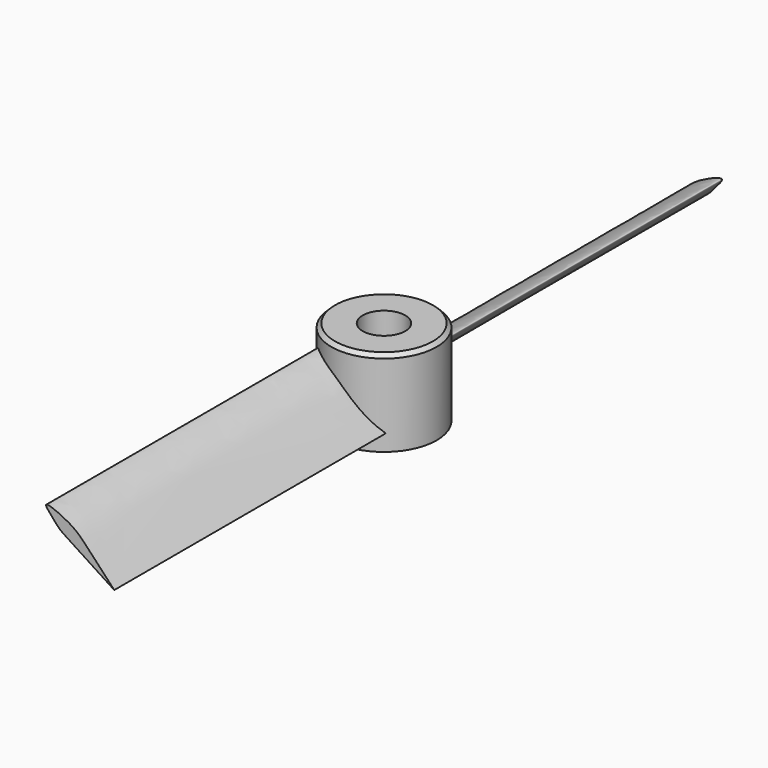
from build123d import *

# Parameters (mm, degrees)
F0_R     = 7.05
F0_R_2   = 2.85
F1_DEPTH = 11.5
F3_DEPTH = 50.8
F4_R     = 5
F6_DEPTH = 50.8
F7_R     = 5
F8_DEPTH = 25
F9_SIZE  = 0.5


# Not quite as in the source:
# - a feature names something its author has since deleted; it is built from what else it names


with BuildPart() as f1:
    # F0 (on Top) → F1 (new body)
    with BuildSketch(Plane.XY):
        Circle(F0_R)
        Circle(F0_R_2, mode=Mode.SUBTRACT)
        Circle(F0_R_2)
    extrude(amount=F1_DEPTH)

    # F2 (on Front) → F3 (join)
    with BuildSketch(Plane.XZ):
        with BuildLine():
            add(Edge.make_bspline(
                [(-2.8507792313, 7.0072189362), (-3.7405771521, 8.1520514624), (-5.7662751539, 10.0693319158), (-1.5520604506, 8.3439902136), (0.1962566258, 6.9176895133), (2.3983110105, 4.4577370851), (3.828236793, 2.9490531221), (4.5479491008, 2.1968713324)],
                knots=[0, 0, 0, 0, 0.1977876363, 0.3919769243, 0.5835513721, 0.7917756861, 1, 1, 1, 1], degree=3))
            Line((-2.8507792313, 7.0072189362), (4.5479491008, 2.1968713324))
        make_face()
    extrude(amount=F3_DEPTH)

    # F4
    f4_edges = [f1.edges().sort_by_distance(p)[0] for p in [
        (-2.850779, -28.623956, 7.007219),
    ]]
    fillet(f4_edges, radius=F4_R)

    # F5 (on Front) → F6 (join)
    with BuildSketch(Plane.XZ):
        with BuildLine():
            Line((-4.5481572581, 2.1965831871), (2.8505710739, 7.0069307909))
            add(Edge.make_bspline(
                [(2.8505710739, 7.0069307909), (3.7403689947, 8.1517633171), (5.7660669965, 10.0690437705), (1.5518522933, 8.3437020683), (-0.1964647831, 6.917401368), (-2.3985191678, 4.4574489398), (-3.8284449503, 2.9487649768), (-4.5481572581, 2.1965831871)],
                knots=[0, 0, 0, 0, 0.1977876363, 0.3919769243, 0.5835513721, 0.7917756861, 1, 1, 1, 1], degree=3))
        make_face()
    extrude(amount=-F6_DEPTH)

    # F7
    f7_edges = [f1.edges().sort_by_distance(p)[0] for p in [
        (2.850571, 28.624002, 7.006931),
    ]]
    fillet(f7_edges, radius=F7_R)

    # F0 (on Top) → F8 (cut)
    with BuildSketch(Plane.XY):
        Circle(F0_R_2)
    extrude(amount=F8_DEPTH, mode=Mode.SUBTRACT)

    # F9
    f9_edges = [f1.edges().sort_by_distance(p)[0] for p in [
        (-7.05, 0, 11.5),
    ]]
    chamfer(f9_edges, length=F9_SIZE)


solid = f1.part
